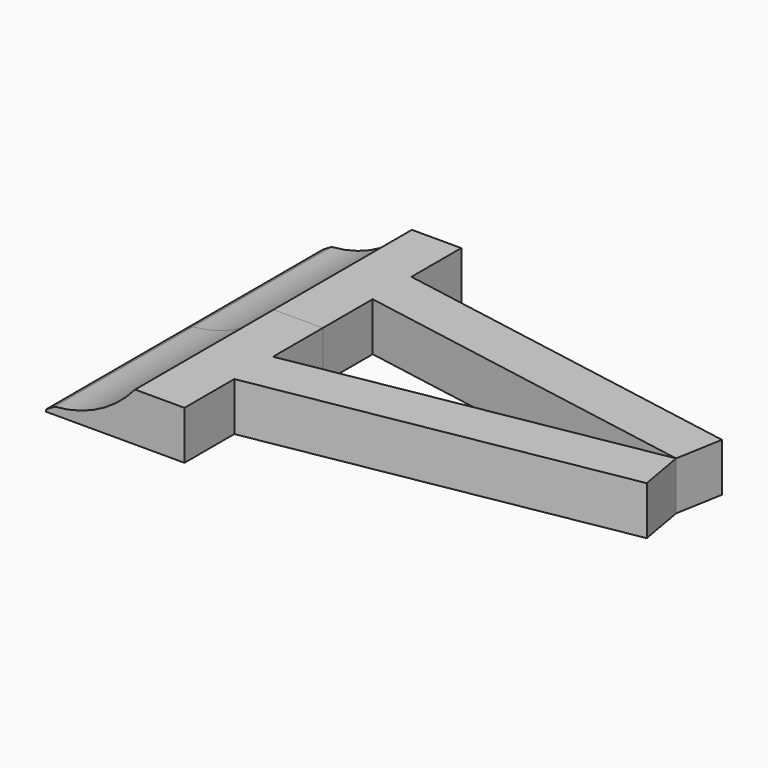
from build123d import *

# Parameters (mm, degrees)
F1_DEPTH    = 25
F2_T1_DEPTH = 31.4504398491
F4_DEPTH    = 7


# Not quite as in the source:
# - a fillet or chamfer that OpenCascade refuses, or shapes differently, is made with other operations: its cross-section is extruded or revolved along the edge and cut away or added


with BuildPart() as f1:
    # F0 (on Front) → F1 (new body)
    with BuildSketch(Plane.XZ):
        with BuildLine():
            Line((0, 1), (0, 0))
            Line((0, 0), (20, 0))
            Line((20, 0), (20, 7))
            Line((20, 7), (12.8650542249, 7))
            ThreePointArc((12.8650542249, 7), (7.09770421, 2.5737434285), (0, 1))
        make_face()
    extrude(amount=F1_DEPTH)

    # F2: chamfer of 0.75 x 1.2990381057 on 1 edges, made by hand

    # F2_s2 → F2_t1 (cut)
    with BuildSketch(Plane.XZ.offset(-3.2252199245)):
        with BuildLine():
            Line((1.2434998223, 1.0461045215), (0, 0.2981636822))
            Line((0, 0.2981636822), (0, 1))
            ThreePointArc((0, 1), (0.6449381871, 1.0123894461), (1.2434998223, 1.0461045215))
        make_face()
    extrude(amount=F2_T1_DEPTH, mode=Mode.SUBTRACT)

    # F3 (on face) → F4 (join, through all)
    with BuildSketch(Plane.XY.offset(7)):
        Polygon((71.0415363766, 0), (20, -9), (20, -16), (72.2386068782, -6.7889241728), align=None)
    extrude(amount=-F4_DEPTH)


with BuildPart() as f5_1:
    # F5: instance of F1
    add(f1.part.mirror(Plane.XZ))


solid = Compound([f1.part, f5_1.part])
